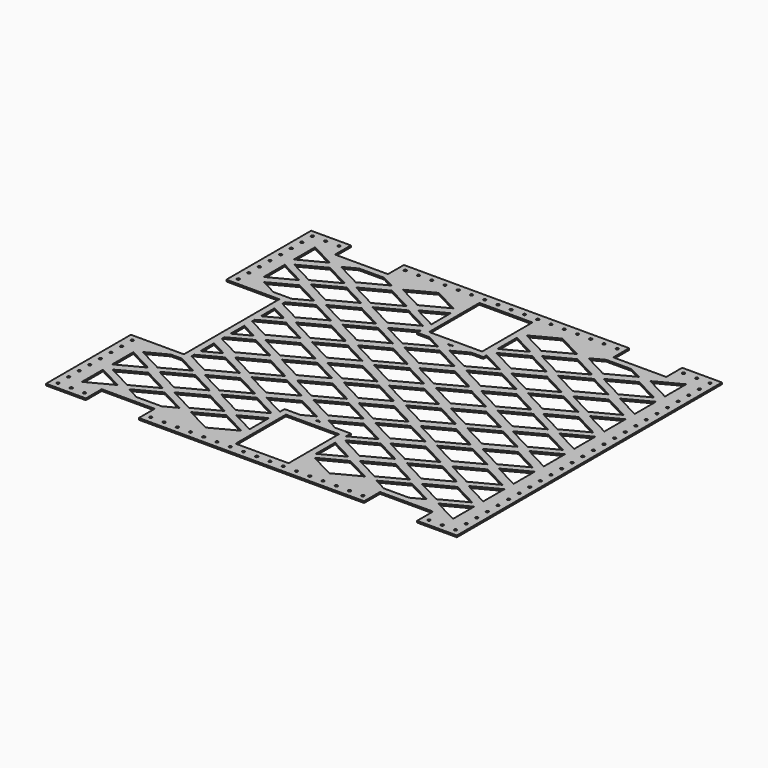
from build123d import *

# Parameters (mm, degrees)
F0_R     = 2.5527
F1_DEPTH = 3.175


# Not quite as in the source:
# - a feature names something its author has since deleted; it is built from what else it names


with BuildPart() as f1:
    # F0 (on Top) → F1 (new body)
    with BuildSketch(Plane.XY):
        with BuildLine():
            Line((76.2, 0), (0, 0))
            Line((0, 0), (0, -190.5))
            Line((0, -190.5), (10.1473, -190.5))
            ThreePointArc((10.1473, -190.5), (12.7, -187.9473), (15.2527, -190.5))
            Line((15.2527, -190.5), (80.0877551055, -190.5))
            Line((80.0877551055, -190.5), (48.9857142864, -174.1714285703))
            Line((48.9857142864, -174.1714285703), (97.3666666684, -148.7714285703))
            Line((97.3666666684, -148.7714285703), (145.7476190503, -174.1714285703))
            Line((145.7476190503, -174.1714285703), (114.3, -190.6814285714))
            Line((114.3, -190.6814285714), (114.3, -205.4678644))
            Line((114.3, -205.4678644), (156.6333333342, -183.2428644))
            Line((156.6333333342, -183.2428644), (205.0142857161, -208.6428644))
            Line((205.0142857161, -208.6428644), (156.6333333342, -234.0428644))
            Line((156.6333333342, -234.0428644), (114.3, -211.8178644))
            Line((114.3, -211.8178644), (114.3, -230.2328571396))
            Line((114.3, -230.2328571396), (145.7476190503, -246.7428571407))
            Line((145.7476190503, -246.7428571407), (114.3, -263.2528571417))
            Line((114.3, -263.2528571417), (114.3, -278.0392966))
            Line((114.3, -278.0392966), (156.6333333342, -255.8142966))
            Line((156.6333333342, -255.8142966), (205.0142857161, -281.2142966))
            Line((205.0142857161, -281.2142966), (156.6333333342, -306.6142966))
            Line((156.6333333342, -306.6142966), (114.3, -284.3892966))
            Line((114.3, -284.3892966), (114.3, -302.80428571))
            Line((114.3, -302.80428571), (145.7476190503, -319.314285711))
            Line((145.7476190503, -319.314285711), (114.3, -335.8242857121))
            Line((114.3, -335.8242857121), (114.3, -350.6107288))
            Line((114.3, -350.6107288), (156.6333333342, -328.3857288))
            Line((156.6333333342, -328.3857288), (205.0142857161, -353.7857288))
            Line((205.0142857161, -353.7857288), (156.6333333342, -379.1857288))
            Line((156.6333333342, -379.1857288), (114.3, -356.9607288))
            Line((114.3, -356.9607288), (114.3, -375.3757142803))
            Line((114.3, -375.3757142803), (145.7476190503, -391.8857142814))
            Line((145.7476190503, -391.8857142814), (114.3, -408.3957142824))
            Line((114.3, -408.3957142824), (114.3, -423.182161))
            Line((114.3, -423.182161), (156.6333333342, -400.957161))
            Line((156.6333333342, -400.957161), (205.0142857161, -426.357161))
            Line((205.0142857161, -426.357161), (156.6333333342, -451.757161))
            Line((156.6333333342, -451.757161), (114.3, -429.532161))
            Line((114.3, -429.532161), (114.3, -444.5))
            Line((114.3, -444.5), (107.7340136177, -444.5))
            Line((107.7340136177, -444.5), (145.7476190503, -464.4571428517))
            Line((145.7476190503, -464.4571428517), (97.3666666684, -489.8571428517))
            Line((97.3666666684, -489.8571428517), (48.9857142864, -464.4571428517))
            Line((48.9857142864, -464.4571428517), (86.999319719, -444.5))
            Line((86.999319719, -444.5), (15.2527, -444.5))
            ThreePointArc((15.2527, -444.5), (12.7, -447.0527), (10.1473, -444.5))
            Line((10.1473, -444.5), (0, -444.5))
            Line((0, -444.5), (0, -635))
            Line((0, -635), (76.2, -635))
            Line((76.2, -635), (76.2, -596.9))
            Line((76.2, -596.9), (156.6333333342, -596.9))
            Line((156.6333333342, -596.9), (177.8, -596.9))
            Line((177.8, -596.9), (177.8, -635))
            Line((177.8, -635), (609.6, -635))
            Line((609.6, -635), (609.6, -596.9))
            Line((609.6, -596.9), (630.7666666709, -596.9))
            Line((630.7666666709, -596.9), (711.2, -596.9))
            Line((711.2, -596.9), (711.2, -635))
            Line((711.2, -635), (787.4, -635))
            Line((787.4, -635), (787.4, -533.4))
            Line((787.4, -533.4), (787.4, -101.6))
            Line((787.4, -101.6), (787.4, 0))
            Line((787.4, 0), (711.2, 0))
            Line((711.2, 0), (711.2, -38.1))
            Line((711.2, -38.1), (630.7666666709, -38.1))
            Line((630.7666666709, -38.1), (609.6, -38.1))
            Line((609.6, -38.1), (609.6, 0))
            Line((609.6, 0), (177.8, 0))
            Line((177.8, 0), (177.8, -38.1))
            Line((177.8, -38.1), (156.6333333342, -38.1))
            Line((156.6333333342, -38.1), (76.2, -38.1))
            Line((76.2, -38.1), (76.2, 0))
        make_face()
        with Locations((12.7, -622.3)):
            Circle(F0_R, mode=Mode.SUBTRACT)
        with Locations((12.7, -596.9)):
            Circle(F0_R, mode=Mode.SUBTRACT)
        with Locations((38.1, -622.3)):
            Circle(F0_R, mode=Mode.SUBTRACT)
        with Locations((63.5, -622.3)):
            Circle(F0_R, mode=Mode.SUBTRACT)
        with Locations((12.7, -571.5)):
            Circle(F0_R, mode=Mode.SUBTRACT)
        Polygon((86.4809523819, -571.4999999924), (38.1, -596.8999999924), (38.1, -546.0999999924), align=None, mode=Mode.SUBTRACT)
        Polygon((180.8238579061, -584.2), (156.6333333342, -596.9000254), (132.4428087623, -584.2), (108.2523809523, -571.5000254), (156.6333333342, -546.1000254), (205.0142857161, -571.5000254), align=None, mode=Mode.SUBTRACT)
        with Locations((12.7, -546.1)):
            Circle(F0_R, mode=Mode.SUBTRACT)
        with Locations((12.7, -520.7)):
            Circle(F0_R, mode=Mode.SUBTRACT)
        with Locations((12.7, -495.3)):
            Circle(F0_R, mode=Mode.SUBTRACT)
        Polygon((86.4809523819, -498.928571422), (38.1, -524.328571422), (38.1, -473.528571422), align=None, mode=Mode.SUBTRACT)
        Polygon((97.3666666684, -562.428571422), (48.9857142864, -537.028571422), (97.3666666684, -511.628571422), (145.7476190503, -537.028571422), align=None, mode=Mode.SUBTRACT)
        Polygon((156.6333333342, -524.3285932), (108.2523809523, -498.9285932), (156.6333333342, -473.5285932), (205.0142857161, -498.9285932), align=None, mode=Mode.SUBTRACT)
        with Locations((190.5, -622.3)):
            Circle(F0_R, mode=Mode.SUBTRACT)
        with Locations((215.9, -622.3)):
            Circle(F0_R, mode=Mode.SUBTRACT)
        with Locations((241.3, -622.3)):
            Circle(F0_R, mode=Mode.SUBTRACT)
        with Locations((266.7, -622.3)):
            Circle(F0_R, mode=Mode.SUBTRACT)
        Polygon((275.1666666684, -596.9000254), (226.7857142864, -571.5000254), (275.1666666684, -546.1000254), (323.5476190503, -571.5000254), align=None, mode=Mode.SUBTRACT)
        with Locations((292.1, -622.3)):
            Circle(F0_R, mode=Mode.SUBTRACT)
        with Locations((317.5, -622.3)):
            Circle(F0_R, mode=Mode.SUBTRACT)
        with Locations((342.9, -622.3)):
            Circle(F0_R, mode=Mode.SUBTRACT)
        with Locations((368.3, -622.3)):
            Circle(F0_R, mode=Mode.SUBTRACT)
        Polygon((215.9000000025, -562.428571422), (167.5190476206, -537.028571422), (215.9000000025, -511.628571422), (264.2809523845, -537.028571422), align=None, mode=Mode.SUBTRACT)
        Polygon((275.1666666684, -524.3285932), (226.7857142864, -498.9285932), (275.1666666684, -473.5285932), (323.5476190503, -498.9285932), align=None, mode=Mode.SUBTRACT)
        with Locations((12.7, -469.9)):
            Circle(F0_R, mode=Mode.SUBTRACT)
        Polygon((215.9000000025, -489.8571428517), (167.5190476206, -464.4571428517), (215.9000000025, -439.0571428517), (264.2809523845, -464.4571428517), align=None, mode=Mode.SUBTRACT)
        Polygon((275.1666666684, -451.757161), (226.7857142864, -426.357161), (275.1666666684, -400.957161), (323.5476190503, -426.357161), align=None, mode=Mode.SUBTRACT)
        Polygon((215.9000000025, -417.2857142814), (167.5190476206, -391.8857142814), (215.9000000025, -366.4857142814), (264.2809523845, -391.8857142814), align=None, mode=Mode.SUBTRACT)
        Polygon((215.9000000025, -344.714285711), (167.5190476206, -319.314285711), (215.9000000025, -293.914285711), (264.2809523845, -319.314285711), align=None, mode=Mode.SUBTRACT)
        Polygon((275.1666666684, -379.1857288), (226.7857142864, -353.7857288), (275.1666666684, -328.3857288), (323.5476190503, -353.7857288), align=None, mode=Mode.SUBTRACT)
        Polygon((334.4333333367, -417.2857142814), (286.0523809548, -391.8857142814), (334.4333333367, -366.4857142814), (382.8142857186, -391.8857142814), align=None, mode=Mode.SUBTRACT)
        Polygon((334.4333333367, -344.714285711), (286.0523809548, -319.314285711), (334.4333333367, -293.914285711), (382.8142857186, -319.314285711), align=None, mode=Mode.SUBTRACT)
        with Locations((393.7, -622.3)):
            Circle(F0_R, mode=Mode.SUBTRACT)
        with Locations((419.1, -622.3)):
            Circle(F0_R, mode=Mode.SUBTRACT)
        with Locations((444.5, -622.3)):
            Circle(F0_R, mode=Mode.SUBTRACT)
        with Locations((469.9, -622.3)):
            Circle(F0_R, mode=Mode.SUBTRACT)
        with Locations((495.3, -622.3)):
            Circle(F0_R, mode=Mode.SUBTRACT)
        with Locations((520.7, -622.3)):
            Circle(F0_R, mode=Mode.SUBTRACT)
        with Locations((546.1, -622.3)):
            Circle(F0_R, mode=Mode.SUBTRACT)
        with Locations((571.5, -622.3)):
            Circle(F0_R, mode=Mode.SUBTRACT)
        Polygon((512.2333333367, -596.9000254), (463.8523809548, -571.5000254), (512.2333333367, -546.1000254), (560.6142857186, -571.5000254), align=None, mode=Mode.SUBTRACT)
        Polygon((457.2, -609.6), (444.5, -609.6), (342.9, -609.6), (330.2, -609.6), (330.2, -560.2060714203), (286.0523809548, -537.028571422), (330.2, -513.8510714238), (330.2, -487.63464285), (286.0523809548, -464.4571428517), (334.4333333367, -439.0571428517), (382.8142857186, -464.4571428517), (360.3517006738, -476.25), (388.5163680024, -476.25), (393.7000000025, -473.5285932), (398.8836320026, -476.25), (427.0482993338, -476.25), (404.585714289, -464.4571428517), (452.9666666709, -439.0571428517), (501.3476190528, -464.4571428517), (457.2, -487.634642854), (457.2, -513.8510714198), (501.3476190528, -537.028571422), (457.2, -560.2060714243), align=None, mode=Mode.SUBTRACT)
        Polygon((571.5000000051, -562.428571422), (523.1190476232, -537.028571422), (571.5000000051, -511.628571422), (619.880952387, -537.028571422), align=None, mode=Mode.SUBTRACT)
        Polygon((512.2333333367, -524.3285932), (463.8523809548, -498.9285932), (512.2333333367, -473.5285932), (560.6142857186, -498.9285932), align=None, mode=Mode.SUBTRACT)
        with Locations((596.9, -622.3)):
            Circle(F0_R, mode=Mode.SUBTRACT)
        Polygon((654.9571912428, -584.2), (630.7666666709, -596.9000254), (606.576142099, -584.2), (582.385714289, -571.5000254), (630.7666666709, -546.1000254), (679.1476190528, -571.5000254), align=None, mode=Mode.SUBTRACT)
        with Locations((723.9, -622.3)):
            Circle(F0_R, mode=Mode.SUBTRACT)
        with Locations((749.3, -622.3)):
            Circle(F0_R, mode=Mode.SUBTRACT)
        with Locations((774.7, -622.3)):
            Circle(F0_R, mode=Mode.SUBTRACT)
        with Locations((774.7, -596.9)):
            Circle(F0_R, mode=Mode.SUBTRACT)
        Polygon((700.9190452, -571.4999999924), (749.3, -546.0999999924), (749.3, -596.8999999924), align=None, mode=Mode.SUBTRACT)
        with Locations((774.7, -571.5)):
            Circle(F0_R, mode=Mode.SUBTRACT)
        Polygon((630.7666666709, -524.3285932), (582.385714289, -498.9285932), (630.7666666709, -473.5285932), (679.1476190528, -498.9285932), align=None, mode=Mode.SUBTRACT)
        Polygon((690.0333333393, -562.428571422), (641.6523809573, -537.028571422), (690.0333333393, -511.628571422), (738.4142857212, -537.028571422), align=None, mode=Mode.SUBTRACT)
        with Locations((774.7, -546.1)):
            Circle(F0_R, mode=Mode.SUBTRACT)
        with Locations((774.7, -520.7)):
            Circle(F0_R, mode=Mode.SUBTRACT)
        Polygon((700.9190452, -498.928571422), (749.3, -473.528571422), (749.3, -524.328571422), align=None, mode=Mode.SUBTRACT)
        with Locations((774.7, -495.3)):
            Circle(F0_R, mode=Mode.SUBTRACT)
        Polygon((393.7000000025, -451.757161), (345.3190476206, -426.357161), (393.7000000025, -400.957161), (442.0809523845, -426.357161), align=None, mode=Mode.SUBTRACT)
        Polygon((571.5000000051, -489.8571428517), (523.1190476232, -464.4571428517), (571.5000000051, -439.0571428517), (619.880952387, -464.4571428517), align=None, mode=Mode.SUBTRACT)
        Polygon((512.2333333367, -451.757161), (463.8523809548, -426.357161), (512.2333333367, -400.957161), (560.6142857186, -426.357161), align=None, mode=Mode.SUBTRACT)
        Polygon((452.9666666709, -417.2857142814), (404.585714289, -391.8857142814), (452.9666666709, -366.4857142814), (501.3476190528, -391.8857142814), align=None, mode=Mode.SUBTRACT)
        Polygon((393.7000000025, -379.1857288), (345.3190476206, -353.7857288), (393.7000000025, -328.3857288), (442.0809523845, -353.7857288), align=None, mode=Mode.SUBTRACT)
        Polygon((452.9666666709, -344.714285711), (404.585714289, -319.314285711), (452.9666666709, -293.914285711), (501.3476190528, -319.314285711), align=None, mode=Mode.SUBTRACT)
        Polygon((571.5000000051, -417.2857142814), (523.1190476232, -391.8857142814), (571.5000000051, -366.4857142814), (619.880952387, -391.8857142814), align=None, mode=Mode.SUBTRACT)
        Polygon((512.2333333367, -379.1857288), (463.8523809548, -353.7857288), (512.2333333367, -328.3857288), (560.6142857186, -353.7857288), align=None, mode=Mode.SUBTRACT)
        Polygon((571.5000000051, -344.714285711), (523.1190476232, -319.314285711), (571.5000000051, -293.914285711), (619.880952387, -319.314285711), align=None, mode=Mode.SUBTRACT)
        Polygon((630.7666666709, -451.757161), (582.385714289, -426.357161), (630.7666666709, -400.957161), (679.1476190528, -426.357161), align=None, mode=Mode.SUBTRACT)
        Polygon((690.0333333393, -489.8571428517), (641.6523809573, -464.4571428517), (690.0333333393, -439.0571428517), (738.4142857212, -464.4571428517), align=None, mode=Mode.SUBTRACT)
        with Locations((774.7, -469.9)):
            Circle(F0_R, mode=Mode.SUBTRACT)
        with Locations((774.7, -444.5)):
            Circle(F0_R, mode=Mode.SUBTRACT)
        Polygon((700.9190452, -426.3571428517), (749.3, -400.9571428517), (749.3, -451.7571428517), align=None, mode=Mode.SUBTRACT)
        with Locations((774.7, -419.1)):
            Circle(F0_R, mode=Mode.SUBTRACT)
        Polygon((630.7666666709, -379.1857288), (582.385714289, -353.7857288), (630.7666666709, -328.3857288), (679.1476190528, -353.7857288), align=None, mode=Mode.SUBTRACT)
        Polygon((690.0333333393, -417.2857142814), (641.6523809573, -391.8857142814), (690.0333333393, -366.4857142814), (738.4142857212, -391.8857142814), align=None, mode=Mode.SUBTRACT)
        with Locations((774.7, -393.7)):
            Circle(F0_R, mode=Mode.SUBTRACT)
        with Locations((774.7, -368.3)):
            Circle(F0_R, mode=Mode.SUBTRACT)
        Polygon((700.9190452, -353.7857142814), (749.3, -328.3857142814), (749.3, -379.1857142814), align=None, mode=Mode.SUBTRACT)
        Polygon((690.0333333393, -344.714285711), (641.6523809573, -319.314285711), (690.0333333393, -293.914285711), (738.4142857212, -319.314285711), align=None, mode=Mode.SUBTRACT)
        with Locations((774.7, -342.9)):
            Circle(F0_R, mode=Mode.SUBTRACT)
        with Locations((12.7, -165.1)):
            Circle(F0_R, mode=Mode.SUBTRACT)
        Polygon((275.1666666684, -306.6142966), (226.7857142864, -281.2142966), (275.1666666684, -255.8142966), (323.5476190503, -281.2142966), align=None, mode=Mode.SUBTRACT)
        Polygon((215.9000000025, -272.1428571407), (167.5190476206, -246.7428571407), (215.9000000025, -221.3428571407), (264.2809523845, -246.7428571407), align=None, mode=Mode.SUBTRACT)
        Polygon((334.4333333367, -272.1428571407), (286.0523809548, -246.7428571407), (334.4333333367, -221.3428571407), (382.8142857186, -246.7428571407), align=None, mode=Mode.SUBTRACT)
        Polygon((275.1666666684, -234.0428644), (226.7857142864, -208.6428644), (275.1666666684, -183.2428644), (323.5476190503, -208.6428644), align=None, mode=Mode.SUBTRACT)
        Polygon((215.9000000025, -199.5714285703), (167.5190476206, -174.1714285703), (215.9000000025, -148.7714285703), (264.2809523845, -174.1714285703), align=None, mode=Mode.SUBTRACT)
        with Locations((12.7, -139.7)):
            Circle(F0_R, mode=Mode.SUBTRACT)
        Polygon((86.4809523819, -136.0714285703), (38.1, -161.4714285703), (38.1, -110.6714285703), align=None, mode=Mode.SUBTRACT)
        with Locations((12.7, -114.3)):
            Circle(F0_R, mode=Mode.SUBTRACT)
        with Locations((12.7, -88.9)):
            Circle(F0_R, mode=Mode.SUBTRACT)
        Polygon((156.6333333342, -161.4714322), (108.2523809523, -136.0714322), (156.6333333342, -110.6714322), (205.0142857161, -136.0714322), align=None, mode=Mode.SUBTRACT)
        Polygon((145.7476190503, -101.6), (97.3666666684, -127), (48.9857142864, -101.6), (97.3666666684, -76.2), align=None, mode=Mode.SUBTRACT)
        with Locations((12.7, -63.5)):
            Circle(F0_R, mode=Mode.SUBTRACT)
        Polygon((38.1, -88.9), (38.1, -38.1), (86.4809523819, -63.5), align=None, mode=Mode.SUBTRACT)
        with Locations((12.7, -38.1)):
            Circle(F0_R, mode=Mode.SUBTRACT)
        with Locations((12.7, -12.7)):
            Circle(F0_R, mode=Mode.SUBTRACT)
        with Locations((38.1, -12.7)):
            Circle(F0_R, mode=Mode.SUBTRACT)
        with Locations((63.5, -12.7)):
            Circle(F0_R, mode=Mode.SUBTRACT)
        Polygon((132.4428571432, -50.8), (156.6333333342, -38.1), (180.8238095251, -50.8), (205.0142857161, -63.5), (156.6333333342, -88.9), (108.2523809523, -63.5), align=None, mode=Mode.SUBTRACT)
        Polygon((275.1666666684, -161.4714322), (226.7857142864, -136.0714322), (275.1666666684, -110.6714322), (323.5476190503, -136.0714322), align=None, mode=Mode.SUBTRACT)
        Polygon((215.9000000025, -127), (167.5190476206, -101.6), (215.9000000025, -76.2), (264.2809523845, -101.6), align=None, mode=Mode.SUBTRACT)
        Polygon((275.1666666684, -88.9), (226.7857142864, -63.5), (275.1666666684, -38.1), (323.5476190503, -63.5), align=None, mode=Mode.SUBTRACT)
        with Locations((190.5, -12.7)):
            Circle(F0_R, mode=Mode.SUBTRACT)
        with Locations((215.9, -12.7)):
            Circle(F0_R, mode=Mode.SUBTRACT)
        with Locations((241.3, -12.7)):
            Circle(F0_R, mode=Mode.SUBTRACT)
        with Locations((266.7, -12.7)):
            Circle(F0_R, mode=Mode.SUBTRACT)
        with Locations((292.1, -12.7)):
            Circle(F0_R, mode=Mode.SUBTRACT)
        with Locations((317.5, -12.7)):
            Circle(F0_R, mode=Mode.SUBTRACT)
        with Locations((342.9, -12.7)):
            Circle(F0_R, mode=Mode.SUBTRACT)
        with Locations((368.3, -12.7)):
            Circle(F0_R, mode=Mode.SUBTRACT)
        Polygon((393.7000000025, -306.6142966), (345.3190476206, -281.2142966), (393.7000000025, -255.8142966), (442.0809523845, -281.2142966), align=None, mode=Mode.SUBTRACT)
        Polygon((452.9666666709, -272.1428571407), (404.585714289, -246.7428571407), (452.9666666709, -221.3428571407), (501.3476190528, -246.7428571407), align=None, mode=Mode.SUBTRACT)
        Polygon((512.2333333367, -306.6142966), (463.8523809548, -281.2142966), (512.2333333367, -255.8142966), (560.6142857186, -281.2142966), align=None, mode=Mode.SUBTRACT)
        Polygon((571.5000000051, -272.1428571407), (523.1190476232, -246.7428571407), (571.5000000051, -221.3428571407), (619.880952387, -246.7428571407), align=None, mode=Mode.SUBTRACT)
        Polygon((393.7000000025, -234.0428644), (345.3190476206, -208.6428644), (393.7000000025, -183.2428644), (442.0809523845, -208.6428644), align=None, mode=Mode.SUBTRACT)
        Polygon((512.2333333367, -234.0428644), (463.8523809548, -208.6428644), (512.2333333367, -183.2428644), (560.6142857186, -208.6428644), align=None, mode=Mode.SUBTRACT)
        Polygon((571.5000000051, -199.5714285703), (523.1190476232, -174.1714285703), (571.5000000051, -148.7714285703), (619.880952387, -174.1714285703), align=None, mode=Mode.SUBTRACT)
        Polygon((630.7666666709, -306.6142966), (582.385714289, -281.2142966), (630.7666666709, -255.8142966), (679.1476190528, -281.2142966), align=None, mode=Mode.SUBTRACT)
        Polygon((700.9190452, -281.214285711), (749.3, -255.814285711), (749.3, -306.614285711), align=None, mode=Mode.SUBTRACT)
        with Locations((774.7, -317.5)):
            Circle(F0_R, mode=Mode.SUBTRACT)
        with Locations((774.7, -292.1)):
            Circle(F0_R, mode=Mode.SUBTRACT)
        Polygon((690.0333333393, -272.1428571407), (641.6523809573, -246.7428571407), (690.0333333393, -221.3428571407), (738.4142857212, -246.7428571407), align=None, mode=Mode.SUBTRACT)
        with Locations((774.7, -266.7)):
            Circle(F0_R, mode=Mode.SUBTRACT)
        with Locations((774.7, -241.3)):
            Circle(F0_R, mode=Mode.SUBTRACT)
        Polygon((630.7666666709, -234.0428644), (582.385714289, -208.6428644), (630.7666666709, -183.2428644), (679.1476190528, -208.6428644), align=None, mode=Mode.SUBTRACT)
        Polygon((700.9190452, -208.6428571407), (749.3, -183.2428571407), (749.3, -234.0428571407), align=None, mode=Mode.SUBTRACT)
        with Locations((774.7, -215.9)):
            Circle(F0_R, mode=Mode.SUBTRACT)
        Polygon((690.0333333393, -199.5714285703), (641.6523809573, -174.1714285703), (690.0333333393, -148.7714285703), (738.4142857212, -174.1714285703), align=None, mode=Mode.SUBTRACT)
        with Locations((774.7, -190.5)):
            Circle(F0_R, mode=Mode.SUBTRACT)
        with Locations((774.7, -165.1)):
            Circle(F0_R, mode=Mode.SUBTRACT)
        Polygon((330.2, -25.4), (342.9, -25.4), (444.5, -25.4), (457.2, -25.4), (457.2, -78.4224999977), (501.3476190528, -101.6), (457.2, -124.7775000023), (457.2, -150.9939285681), (501.3476190528, -174.1714285703), (452.9666666709, -199.5714285703), (404.585714289, -174.1714285703), (433.9598639474, -158.75), (398.8836803836, -158.75), (393.7000000025, -161.4714322), (388.5163196215, -158.75), (353.4401360603, -158.75), (382.8142857186, -174.1714285703), (334.4333333367, -199.5714285703), (286.0523809548, -174.1714285703), (330.2, -150.9939285721), (330.2, -124.7774999983), (286.0523809548, -101.6), (330.2, -78.4225000017), align=None, mode=Mode.SUBTRACT)
        Polygon((512.2333333367, -161.4714322), (463.8523809548, -136.0714322), (512.2333333367, -110.6714322), (560.6142857186, -136.0714322), align=None, mode=Mode.SUBTRACT)
        Polygon((571.5000000051, -127), (523.1190476232, -101.6), (571.5000000051, -76.2), (619.880952387, -101.6), align=None, mode=Mode.SUBTRACT)
        with Locations((393.7, -12.7)):
            Circle(F0_R, mode=Mode.SUBTRACT)
        with Locations((419.1, -12.7)):
            Circle(F0_R, mode=Mode.SUBTRACT)
        with Locations((444.5, -12.7)):
            Circle(F0_R, mode=Mode.SUBTRACT)
        with Locations((469.9, -12.7)):
            Circle(F0_R, mode=Mode.SUBTRACT)
        Polygon((512.2333333367, -88.9), (463.8523809548, -63.5), (512.2333333367, -38.1), (560.6142857186, -63.5), align=None, mode=Mode.SUBTRACT)
        with Locations((495.3, -12.7)):
            Circle(F0_R, mode=Mode.SUBTRACT)
        with Locations((520.7, -12.7)):
            Circle(F0_R, mode=Mode.SUBTRACT)
        with Locations((546.1, -12.7)):
            Circle(F0_R, mode=Mode.SUBTRACT)
        with Locations((571.5, -12.7)):
            Circle(F0_R, mode=Mode.SUBTRACT)
        Polygon((630.7666666709, -161.4714322), (582.385714289, -136.0714322), (630.7666666709, -110.6714322), (679.1476190528, -136.0714322), align=None, mode=Mode.SUBTRACT)
        Polygon((700.9190452, -136.0714285703), (749.3, -110.6714285703), (749.3, -161.4714285703), align=None, mode=Mode.SUBTRACT)
        with Locations((774.7, -139.7)):
            Circle(F0_R, mode=Mode.SUBTRACT)
        Polygon((690.0333333393, -127), (641.6523809573, -101.6), (690.0333333393, -76.2), (738.4142857212, -101.6), align=None, mode=Mode.SUBTRACT)
        with Locations((774.7, -114.3)):
            Circle(F0_R, mode=Mode.SUBTRACT)
        with Locations((774.7, -88.9)):
            Circle(F0_R, mode=Mode.SUBTRACT)
        Polygon((606.5761904799, -50.8), (630.7666666709, -38.1), (654.9571428619, -50.8), (679.1476190528, -63.5), (630.7666666709, -88.9), (582.385714289, -63.5), align=None, mode=Mode.SUBTRACT)
        with Locations((596.9, -12.7)):
            Circle(F0_R, mode=Mode.SUBTRACT)
        Polygon((700.9190452, -63.5), (749.3, -38.1), (749.3, -88.9), align=None, mode=Mode.SUBTRACT)
        with Locations((774.7, -63.5)):
            Circle(F0_R, mode=Mode.SUBTRACT)
        with Locations((723.9, -12.7)):
            Circle(F0_R, mode=Mode.SUBTRACT)
        with Locations((774.7, -38.1)):
            Circle(F0_R, mode=Mode.SUBTRACT)
        with Locations((749.3, -12.7)):
            Circle(F0_R, mode=Mode.SUBTRACT)
        with Locations((774.7, -12.7)):
            Circle(F0_R, mode=Mode.SUBTRACT)
        Polygon((457.2, -25.4), (444.5, -25.4), (444.5, -146.05), (423.0741565746, -146.05), (398.8836803836, -158.75), (433.9598639474, -158.75), (452.9666666709, -148.7714285703), (457.2, -150.9939285681), (457.2, -124.7775000023), (457.2, -78.4224999977), align=None)
        with BuildLine():
            Line((101.6, -431.8), (0, -431.8))
            Line((0, -431.8), (0, -444.5))
            Line((0, -444.5), (10.1473, -444.5))
            ThreePointArc((10.1473, -444.5), (12.7, -441.9473), (15.2527, -444.5))
            Line((15.2527, -444.5), (86.999319719, -444.5))
            Line((86.999319719, -444.5), (97.3666666684, -439.0571428517))
            Line((97.3666666684, -439.0571428517), (107.7340136177, -444.5))
            Line((107.7340136177, -444.5), (114.3, -444.5))
            Line((114.3, -444.5), (114.3, -429.532161))
            Line((114.3, -429.532161), (108.2523809523, -426.357161))
            Line((108.2523809523, -426.357161), (114.3, -423.182161))
            Line((114.3, -423.182161), (114.3, -408.3957142824))
            Line((114.3, -408.3957142824), (101.6, -415.0632142823))
            Line((101.6, -415.0632142823), (101.6, -431.8))
        make_face()
        with BuildLine():
            Line((10.1473, -190.5), (0, -190.5))
            Line((0, -190.5), (0, -203.2))
            Line((0, -203.2), (101.6, -203.2))
            Line((101.6, -203.2), (101.6, -223.5653571397))
            Line((101.6, -223.5653571397), (114.3, -230.2328571396))
            Line((114.3, -230.2328571396), (114.3, -211.8178644))
            Line((114.3, -211.8178644), (108.2523809523, -208.6428644))
            Line((108.2523809523, -208.6428644), (114.3, -205.4678644))
            Line((114.3, -205.4678644), (114.3, -190.6814285714))
            Line((114.3, -190.6814285714), (97.3666666684, -199.5714285703))
            Line((97.3666666684, -199.5714285703), (80.0877551055, -190.5))
            Line((80.0877551055, -190.5), (15.2527, -190.5))
            ThreePointArc((15.2527, -190.5), (12.7, -193.0527), (10.1473, -190.5))
        make_face()
        Polygon((342.9, -146.05), (342.9, -122.5550000019), (334.4333333367, -127), (330.2, -124.7774999983), (330.2, -150.9939285721), (334.4333333367, -148.7714285703), (353.4401360603, -158.75), (388.5163196215, -158.75), (364.3258434305, -146.05), align=None)
        Polygon((334.4333333367, -511.628571422), (342.9, -516.0735714202), (342.9, -488.95), (364.3258918115, -488.95), (388.5163680024, -476.25), (360.3517006738, -476.25), (334.4333333367, -489.8571428517), (330.2, -487.63464285), (330.2, -513.8510714238), align=None)
        Polygon((444.5, -488.95), (444.5, -516.0735714242), (452.9666666709, -511.628571422), (457.2, -513.8510714198), (457.2, -487.634642854), (452.9666666709, -489.8571428517), (427.0482993338, -476.25), (398.8836320026, -476.25), (423.0741081936, -488.95), align=None)
        Polygon((342.9, -80.6449999981), (342.9, -25.4), (330.2, -25.4), (330.2, -78.4225000017), (334.4333333367, -76.2), align=None)
        Polygon((330.2, -609.6), (342.9, -609.6), (342.9, -557.9835714239), (334.4333333367, -562.428571422), (330.2, -560.2060714203), align=None)
        Polygon((444.5, -557.9835714199), (444.5, -609.6), (457.2, -609.6), (457.2, -560.2060714243), (452.9666666709, -562.428571422), align=None)
        Polygon((342.9, -122.5550000019), (342.9, -80.6449999981), (334.4333333367, -76.2), (330.2, -78.4225000017), (330.2, -124.7774999983), (334.4333333367, -127), align=None)
        Polygon((334.4333333367, -562.428571422), (342.9, -557.9835714239), (342.9, -516.0735714202), (334.4333333367, -511.628571422), (330.2, -513.8510714238), (330.2, -560.2060714203), align=None)
        Polygon((444.5, -516.0735714242), (444.5, -557.9835714199), (452.9666666709, -562.428571422), (457.2, -560.2060714243), (457.2, -513.8510714198), (452.9666666709, -511.628571422), align=None)
        Polygon((114.3, -230.2328571396), (101.6, -223.5653571397), (101.6, -269.9203571416), (114.3, -263.2528571417), align=None)
        Polygon((114.3, -302.80428571), (101.6, -296.1367857101), (101.6, -342.491785712), (114.3, -335.8242857121), align=None)
        Polygon((101.6, -368.7082142804), (101.6, -415.0632142823), (114.3, -408.3957142824), (114.3, -375.3757142803), align=None)
        Polygon((398.8836803836, -158.75), (423.0741565746, -146.05), (364.3258434305, -146.05), (388.5163196215, -158.75), align=None)
        Polygon((364.3258918115, -488.95), (423.0741081936, -488.95), (398.8836320026, -476.25), (388.5163680024, -476.25), align=None)
        Polygon((114.3, -263.2528571417), (101.6, -269.9203571416), (101.6, -296.1367857101), (114.3, -302.80428571), (114.3, -284.3892966), (108.2523809523, -281.2142966), (114.3, -278.0392966), align=None)
        Polygon((101.6, -342.491785712), (101.6, -368.7082142804), (114.3, -375.3757142803), (114.3, -356.9607288), (108.2523809523, -353.7857288), (114.3, -350.6107288), (114.3, -335.8242857121), align=None)
        Polygon((606.576142099, -584.2), (630.7666666709, -596.9000254), (654.9571912428, -584.2), align=None)
        Polygon((132.4428087623, -584.2), (156.6333333342, -596.9000254), (180.8238579061, -584.2), align=None)
        Polygon((654.9571428619, -50.8), (630.7666666709, -38.1), (606.5761904799, -50.8), align=None)
        Polygon((330.2, -476.25), (330.2, -487.63464285), (334.4333333367, -489.8571428517), (360.3517006738, -476.25), align=None)
        Polygon((452.9666666709, -489.8571428517), (457.2, -487.634642854), (457.2, -476.25), (427.0482993338, -476.25), align=None)
        Polygon((114.3, -190.5), (80.0877551055, -190.5), (97.3666666684, -199.5714285703), (114.3, -190.6814285714), align=None)
        Polygon((156.6333333342, -50.8), (156.6333333342, -38.1), (132.4428571432, -50.8), align=None)
        Polygon((180.8238095251, -50.8), (156.6333333342, -38.1), (156.6333333342, -50.8), align=None)
        Polygon((334.4333333367, -148.7714285703), (330.2, -150.9939285721), (330.2, -158.75), (353.4401360603, -158.75), align=None)
        Polygon((452.9666666709, -148.7714285703), (433.9598639474, -158.75), (457.2, -158.75), (457.2, -150.9939285681), align=None)
        Polygon((97.3666666684, -439.0571428517), (86.999319719, -444.5), (107.7340136177, -444.5), align=None)
        Polygon((108.2523809523, -208.6428644), (114.3, -211.8178644), (114.3, -205.4678644), align=None)
        Polygon((108.2523809523, -353.7857288), (114.3, -356.9607288), (114.3, -350.6107288), align=None)
        Polygon((114.3, -284.3892966), (114.3, -278.0392966), (108.2523809523, -281.2142966), align=None)
        Polygon((114.3, -429.532161), (114.3, -423.182161), (108.2523809523, -426.357161), align=None)
    extrude(amount=F1_DEPTH)


solid = f1.part
